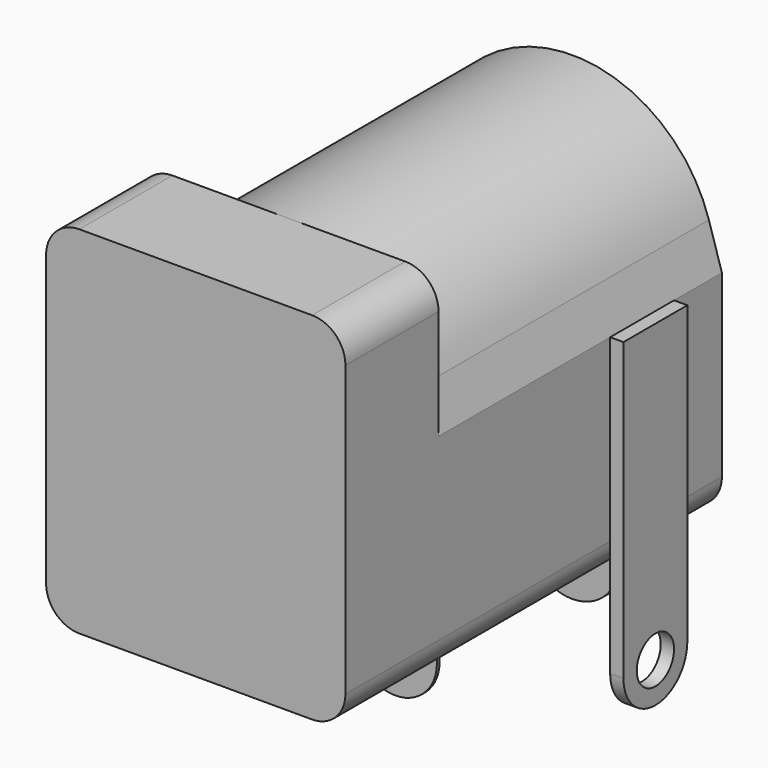
from build123d import *

# Parameters (mm, degrees)
F1_DEPTH  = 10.65
F2_W      = 9
F2_H      = 10.7
F3_DEPTH  = 3.5
F4_R      = 1
F5_R      = 0.7
F6_DEPTH  = 0.4
F7_R      = 0.7
F8_DEPTH  = 0.4
F10_R     = 0.7
F11_DEPTH = 0.05


with BuildPart() as f1:
    # F0 (on Front) → F1 (new body)
    with BuildSketch(Plane.XZ):
        with BuildLine():
            ThreePointArc((4.1088888889, 1.2676876976), (0, 4.3), (-4.1088888889, 1.2676876976))
            Line((-4.1088888889, 1.2676876976), (-4.5, 0))
            Line((-4.5, 0), (-4.5, -6.4))
            Line((-4.5, -6.4), (0, -6.4))
            Line((0, -6.4), (4.5, -6.4))
            Line((4.5, -6.4), (4.5, 0))
            Line((4.5, 0), (4.1088888889, 1.2676876976))
        make_face()
    extrude(amount=-F1_DEPTH)

    # F2 (on face) → F3 (join)
    with BuildSketch(Plane.XZ):
        with Locations((0, -1.05)):
            Rectangle(F2_W, F2_H)
    extrude(amount=F3_DEPTH)

    # F4
    f4_edges = [f1.edges().sort_by_distance(p)[0] for p in [
        (4.5, -1.75, 4.3),
        (-4.5, -1.75, 4.3),
        (4.5, 3.575, -6.4),
        (-4.5, 3.575, -6.4),
    ]]
    fillet(f4_edges, radius=F4_R)

    # F5 (on face) → F6 (join)
    with BuildSketch(Plane.YZ.offset(4.5)):
        with BuildLine():
            ThreePointArc((6.45, -8.9), (7.65, -10.1), (8.85, -8.9))
            Line((8.85, -8.9), (8.85, 0))
            Line((8.85, 0), (6.45, 0))
            Line((6.45, 0), (6.45, -8.9))
        make_face()
        with Locations((7.65, -8.9)):
            Circle(F5_R, mode=Mode.SUBTRACT)
    extrude(amount=F6_DEPTH)

    # F7 (on face) → F8 (join)
    with BuildSketch(Plane(origin=(0, 10.65, 0), x_dir=(-1, 0, 0), z_dir=(0, 1, 0))):
        with BuildLine():
            ThreePointArc((-1.4, -8.7), (0, -10.1), (1.4, -8.7))
            Line((1.4, -8.7), (1.4, 0))
            Line((1.4, 0), (-1.4, 0))
            Line((-1.4, 0), (-1.4, -8.7))
        make_face()
        with Locations((0, -8.7)):
            Circle(F7_R, mode=Mode.SUBTRACT)
    extrude(amount=F8_DEPTH)

    # F10 (on offset) → F11 (join, symmetric)
    with BuildSketch(Plane.XZ.offset(-4.05)):
        with BuildLine():
            ThreePointArc((-1.25, -8.7), (0, -9.95), (1.25, -8.7))
            Line((1.25, -8.7), (1.25, 0))
            Line((1.25, 0), (-1.25, 0))
            Line((-1.25, 0), (-1.25, -8.7))
        make_face()
        with Locations((0, -8.7)):
            Circle(F10_R, mode=Mode.SUBTRACT)
    extrude(amount=F11_DEPTH, both=True)


solid = f1.part
